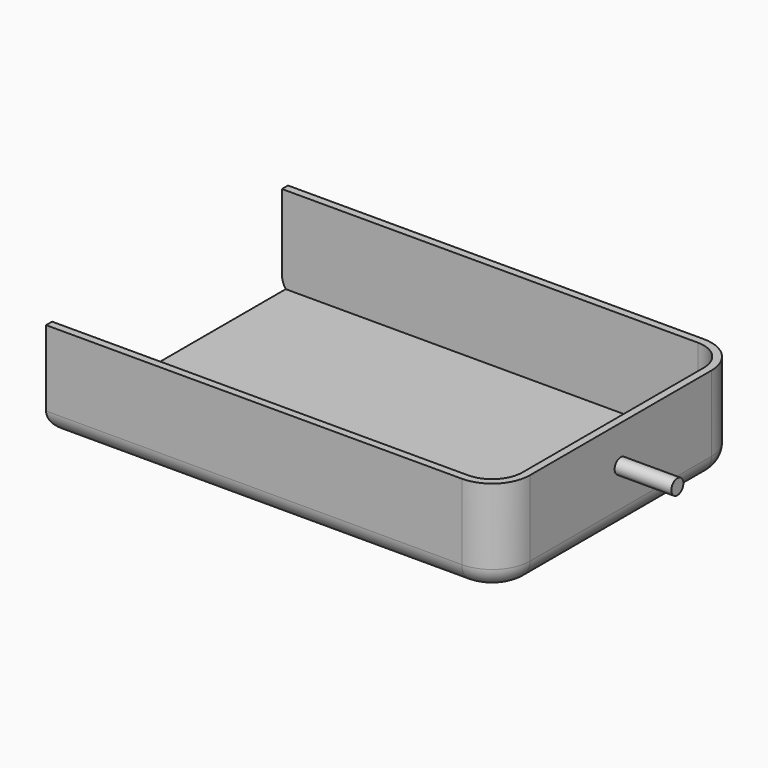
from build123d import *

# Parameters (mm, degrees)
F1_DEPTH     = 63.5
F2_T         = -5.08
F3_R         = 5.08
F4_DEPTH     = 38.1
F5_T1_DEPTH  = 311.15
F5_T3_DEPTH  = 266.7
F5_T5_DEPTH  = 152.4
F5_T8_ANGLE  = 90
F5_T10_ANGLE = 90


# Not quite as in the source:
# - a fillet or chamfer that OpenCascade refuses, or shapes differently, is made with other operations: its cross-section is extruded or revolved along the edge and cut away or added


with BuildPart() as f1:
    # F0 (on Top) → F1 (new body)
    with BuildSketch(Plane.XY):
        with BuildLine():
            Line((-344.2945734978, 176.2892417401), (-401.1594021572, 176.2892417401))
            Line((-401.1594021572, 176.2892417401), (-401.1594021572, -26.9107582599))
            Line((-401.1594021572, -26.9107582599), (-344.2945734978, -26.9107582599))
            Line((-344.2945734978, -26.9107582599), (-121.7594021572, -26.9107582599))
            ThreePointArc((-121.7594021572, -26.9107582599), (-103.7988899151, -19.471270502), (-96.3594021572, -1.5107582599))
            Line((-96.3594021572, -1.5107582599), (-96.3594021572, 6.5090437472))
            Line((-96.3594021572, 6.5090437472), (-96.3594021572, 44.6090437472))
            Line((-96.3594021572, 44.6090437472), (-96.3594021572, 150.8892417401))
            ThreePointArc((-96.3594021572, 150.8892417401), (-103.7988899151, 168.8497539822), (-121.7594021572, 176.2892417401))
            Line((-121.7594021572, 176.2892417401), (-344.2945734978, 176.2892417401))
        make_face()
    extrude(amount=F1_DEPTH)

    # F2
    f2_openings = [f1.faces().sort_by_distance(p)[0] for p in [
        (-249.418343, 74.689242, 63.5),
        (-401.159402, 74.689242, 31.75),
    ]]
    offset(amount=F2_T, openings=f2_openings)

    # F3 (on face) → F4 (join)
    with BuildSketch(Plane.YZ.offset(-96.3594021572)):
        with Locations((74.6892417401, 38.1)):
            Circle(F3_R)
    extrude(amount=F4_DEPTH)

    # F5: fillet of radius 12.7 on 6 edges, made by hand

    # F5_s2 → F5_t1 (cut)
    with BuildSketch(Plane.YZ.offset(-432.9094021572)):
        with BuildLine():
            ThreePointArc((176.2892417401, 12.7), (172.5694978612, 3.7197438789), (163.5892417401, 0))
            Line((163.5892417401, 0), (176.2892417401, 0))
            Line((176.2892417401, 0), (176.2892417401, 12.7))
        make_face()
        with BuildLine():
            ThreePointArc((-14.2107582599, 0), (-23.191014381, 3.7197438789), (-26.9107582599, 12.7))
            Line((-26.9107582599, 12.7), (-26.9107582599, 0))
            Line((-26.9107582599, 0), (-14.2107582599, 0))
        make_face()
    extrude(amount=F5_T1_DEPTH, mode=Mode.SUBTRACT)

    # F5_s4 → F5_t3 (cut)
    with BuildSketch(Plane.XZ.offset(-208.0392417401)):
        with BuildLine():
            ThreePointArc((-401.1594021572, 12.7), (-397.4396582783, 3.7197438789), (-388.4594021572, 0))
            Line((-388.4594021572, 0), (-401.1594021572, 0))
            Line((-401.1594021572, 0), (-401.1594021572, 12.7))
        make_face()
    extrude(amount=F5_T3_DEPTH, mode=Mode.SUBTRACT)

    # F5_s6 → F5_t5 (cut)
    with BuildSketch(Plane.XZ.offset(-150.8892417401)):
        with BuildLine():
            ThreePointArc((-109.0594021572, 0), (-100.0791460361, 3.7197438789), (-96.3594021572, 12.7))
            Line((-96.3594021572, 12.7), (-96.3594021572, 0))
            Line((-96.3594021572, 0), (-109.0594021572, 0))
        make_face()
    extrude(amount=F5_T5_DEPTH, mode=Mode.SUBTRACT)

    # F5_s7 → F5_t8 (revolve, cut)
    with BuildSketch(Plane.YZ.offset(-121.7594021572)):
        with BuildLine():
            ThreePointArc((-14.2107582599, 0), (-23.191014381, 3.7197438789), (-26.9107582599, 12.7))
            Line((-26.9107582599, 12.7), (-26.9107582599, 0))
            Line((-26.9107582599, 0), (-14.2107582599, 0))
        make_face()
    revolve(axis=Axis((-121.7594021572, -1.5107582599, 0), (0, 0, 1)), revolution_arc=F5_T8_ANGLE, mode=Mode.SUBTRACT)

    # F5_s9 → F5_t10 (revolve, cut)
    with BuildSketch(Plane.XZ.offset(-150.8892417401)):
        with BuildLine():
            ThreePointArc((-96.3594021572, 12.7), (-100.0791460361, 3.7197438789), (-109.0594021572, 0))
            Line((-109.0594021572, 0), (-96.3594021572, 0))
            Line((-96.3594021572, 0), (-96.3594021572, 12.7))
        make_face()
    revolve(axis=Axis((-121.7594021572, 150.8892417401, 0), (0, 0, 1)), revolution_arc=F5_T10_ANGLE, mode=Mode.SUBTRACT)


solid = f1.part
